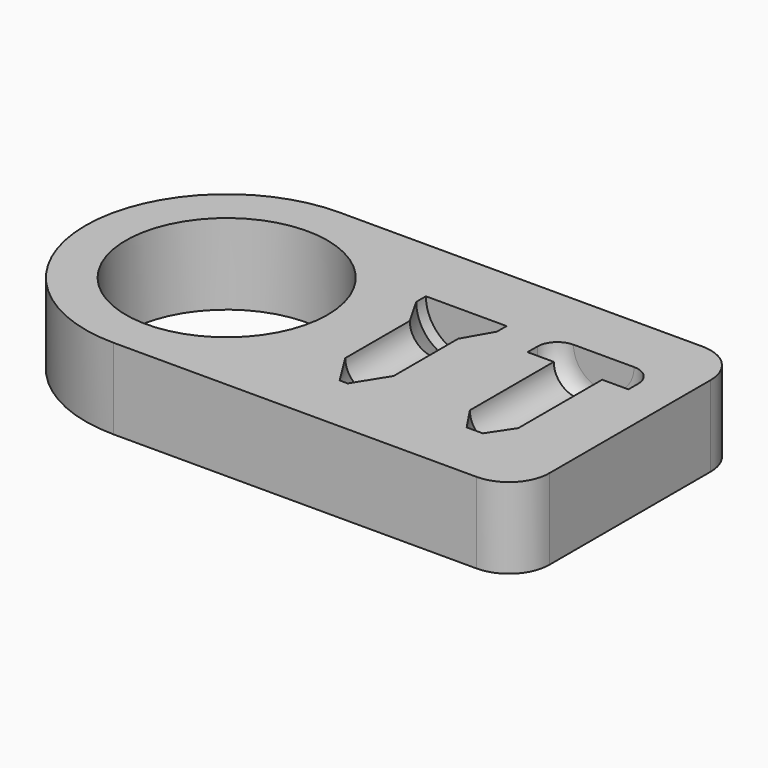
from build123d import *

# Parameters (mm, degrees)
F0_R         = 12.5
F1_DEPTH     = 10
F5_TEXT_SIZE = 5.5555555556
F6_DEPTH     = 1


# Not quite as in the source:
# - Text() gives the source's letters only with a copy of the font that has no kerning and outlines rounded to 1/6400 em; it was checked with that copy


with BuildPart() as f1:
    # F0 (on Top) → F1 (new body)
    with BuildSketch(Plane.XY):
        with BuildLine():
            ThreePointArc((0, 17.5), (5.1256313292, 5.1256313292), (17.5, 0))
            Line((17.5, 0), (62.5, 0))
            ThreePointArc((62.5, 0), (66.0355339059, 1.4644660941), (67.5, 5))
            Line((67.5, 5), (67.5, 30))
            ThreePointArc((67.5, 30), (66.0355339059, 33.5355339059), (62.5, 35))
            Line((62.5, 35), (17.5, 35))
            ThreePointArc((17.5, 35), (5.1256313292, 29.8743686708), (0, 17.5))
        make_face()
        with Locations((17.5, 17.5)):
            Circle(F0_R, mode=Mode.SUBTRACT)
    extrude(amount=F1_DEPTH)

    # F2 (on face) → F3 (revolve, cut)
    with BuildSketch(Plane.XY.offset(10)):
        Polygon((40, 26.5), (40, 7.5), (40.5, 7.5), (43, 11.5), (43, 21.5), (45, 25), (45, 26.5), align=None)
    revolve(axis=Axis((40, 17, 10), (0, 1, 0)), mode=Mode.SUBTRACT)

    # F2 (on face) → F4 (revolve, cut)
    with BuildSketch(Plane.XY.offset(10)):
        with BuildLine():
            Line((56.25, 23.5), (56.25, 7.5))
            Line((56.25, 7.5), (57.25, 7.5))
            Line((57.25, 7.5), (59.25, 10.5))
            Line((59.25, 10.5), (59.25, 23.5))
            Line((59.25, 23.5), (62.5, 23.5))
            Line((62.5, 23.5), (62.5, 25))
            ThreePointArc((62.5, 25), (61.767766953, 26.767766953), (60, 27.5))
            Line((60, 27.5), (56.25, 27.5))
            Line((56.25, 27.5), (56.25, 23.5))
        make_face()
    revolve(axis=Axis((56.25, 15.5, 10), (0, 1, 0)), mode=Mode.SUBTRACT)

    # F5 (on face) → F6 (cut)
    with BuildSketch(Plane(origin=(0, 0, 0), x_dir=(1, 0, 0), z_dir=(0, 0, -1))):
        with Locations((30, -9)):
            Text('1024, 1025', F5_TEXT_SIZE, font='Open Sans', text_align=(TextAlign.LEFT, TextAlign.BOTTOM))
    extrude(amount=-F6_DEPTH, mode=Mode.SUBTRACT)


solid = f1.part
